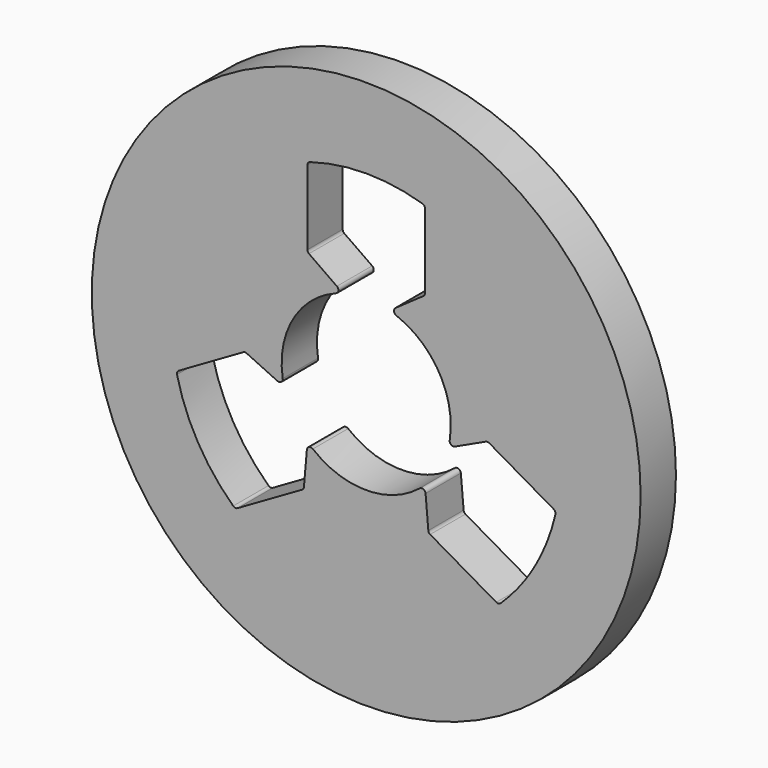
from build123d import *

# Parameters (mm, degrees)
F0_R     = 37.3207707479
F1_DEPTH = 6
F2_R     = 0.5


# Not quite as in the source:
# - two fillets or chamfers of one size are made in one step


with BuildPart() as f1:
    # F0 (on Front) → F1 (new body)
    with BuildSketch(Plane.XZ):
        Circle(F0_R)
        with BuildLine():
            ThreePointArc((-11.1602745113, -2.7745761537), (-9.9592921435, 5.75), (-3.1772838218, 11.0523693168))
            Line((-3.1772838218, 11.0523693168), (-8, 14.4292715395))
            Line((-8, 14.4292715395), (-8, 25.1894103565))
            ThreePointArc((-8, 25.1894103565), (0, 26.4292715395), (8, 25.1894103565))
            Line((8, 25.1894103565), (8, 14.4292715395))
            Line((8, 14.4292715395), (3.1772838218, 11.0523693168))
            ThreePointArc((3.1772838218, 11.0523693168), (9.9592921435, 5.75), (11.1602745113, -2.7745761537))
            Line((11.1602745113, -2.7745761537), (16.4961157113, -0.2864325395))
            Line((16.4961157113, -0.2864325395), (25.8146692751, -5.666501948))
            ThreePointArc((25.8146692751, -5.666501948), (24.9687771204, -8.6640962149), (23.7761097196, -11.5413604358))
            ThreePointArc((23.7761097196, -11.5413604358), (22.7401432363, -13.4681951166), (21.5483693449, -15.3027504941))
            ThreePointArc((21.5483693449, -15.3027504941), (19.880834384, -17.4143279602), (18.0072512686, -19.3454205397))
            Line((18.0072512686, -19.3454205397), (8.4695163323, -13.8388067068))
            Line((8.4695163323, -13.8388067068), (7.9829906895, -8.2777931631))
            ThreePointArc((7.9829906895, -8.2777931631), (0, -11.5), (-7.9829906895, -8.2777931631))
            Line((-7.9829906895, -8.2777931631), (-8.4961157113, -14.142839))
            Line((-8.4961157113, -14.142839), (-17.8146692751, -19.5229084085))
            ThreePointArc((-17.8146692751, -19.5229084085), (-22.8884205567, -13.2146357697), (-25.8146692751, -5.666501948))
            Line((-25.8146692751, -5.666501948), (-16.4961157113, -0.2864325395))
            Line((-16.4961157113, -0.2864325395), (-11.1602745113, -2.7745761537))
        make_face(mode=Mode.SUBTRACT)
    extrude(amount=F1_DEPTH)

    # F2
    f2_edges = [f1.edges().sort_by_distance(p)[0] for p in [
        (-17.814669, -3, -19.522908),
        (-25.814669, -3, -5.666502),
        (-8.496116, -3, -14.142839),
        (-7.982991, -3, -8.277793),
        (7.982991, -3, -8.277793),
        (8.469516, -3, -13.838807),
        (18.007251, -3, -19.345421),
        (25.814669, -3, -5.666502),
        (16.496116, -3, -0.286433),
        (11.160275, -3, -2.774576),
        (3.177284, -3, 11.052369),
        (8, -3, 14.429272),
        (8, -3, 25.18941),
        (-8, -3, 25.18941),
        (-8, -3, 14.429272),
        (-3.177284, -3, 11.052369),
        (-11.160275, -3, -2.774576),
        (-16.496116, -3, -0.286433),
    ]]
    fillet(f2_edges, radius=F2_R)


solid = f1.part
